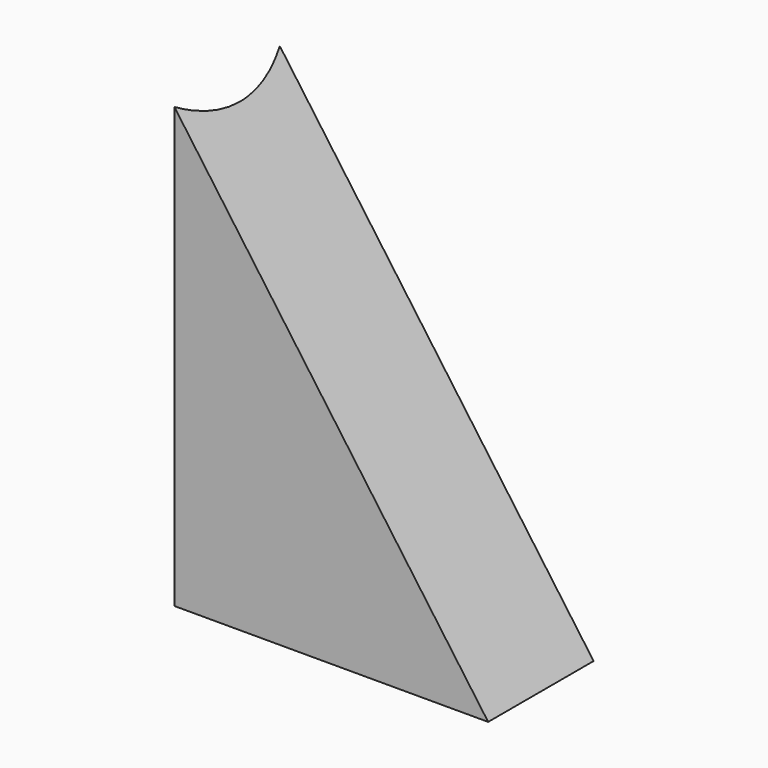
from build123d import *

# Parameters (mm, degrees)
F0_W     = 14.2837
F0_H     = 6
F1_DEPTH = 20
F2_SIZE2 = 14.28369
F2_SIZE  = 19.99999
F4_DEPTH = 25


# Not quite as in the source:
# - a fillet or chamfer is up to 0.001 mm smaller than in the source, because OpenCascade refuses the exact size


with BuildPart() as f1:
    # F0 (on Top) → F1 (new body)
    with BuildSketch(Plane.XY):
        Rectangle(F0_W, F0_H)
    extrude(amount=F1_DEPTH)

    # F2 (size 20 and 14.2837 in the source; OpenCascade refuses exactly that, so slightly less here)
    f2_edges = [f1.edges().sort_by_distance(p)[0] for p in [
        (7.14185, 0, 20),
    ]]
    f2_side = f1.faces().sort_by_distance((7.14185, 0, 10))[0]
    chamfer(f2_edges, length=F2_SIZE, length2=F2_SIZE2, reference=f2_side)

    # F3 (on Top) → F4 (cut)
    with BuildSketch(Plane.XY):
        with BuildLine():
            ThreePointArc((-7.14185, 3), (-22.5580484871, 0), (-7.14185, -3))
            Line((-7.14185, -3), (-7.14185, 3))
        make_face()
        with BuildLine():
            Line((-7.14185, 3), (-7.14185, -3))
            ThreePointArc((-7.14185, -3), (-6.7053550671, -1.5281380997), (-6.5580484871, 0))
            ThreePointArc((-6.5580484871, 0), (-6.7053550671, 1.5281380997), (-7.14185, 3))
        make_face()
    extrude(amount=F4_DEPTH, mode=Mode.SUBTRACT)


solid = f1.part
